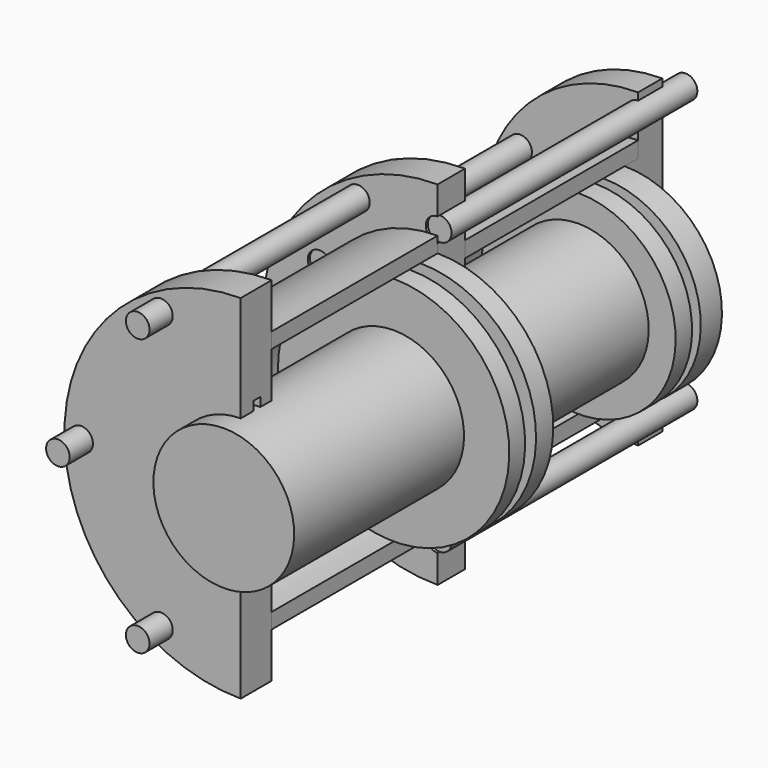
from build123d import *

# Parameters (mm, degrees)
F0_W           = 15.1666663587
F0_H           = 11.4706810564
F8_R           = 3.2667249977
F9_DEPTH       = 77.4214528501
F10_R          = 3.2594816629
F11_DEPTH      = 77.3061978245
F12_DEPTH      = 8
F12_DEPTH_BACK = 83
F13_COUNT      = 6
F14_DEPTH      = 8
F14_DEPTH_BACK = 76.7
F15_COUNT      = 6
F16_W          = 57.5555562973
F16_H          = 106.7500039935
F17_DEPTH      = 100.5891192088
F17_DEPTH_BACK = 60.6954473386


with BuildPart() as f1:
    # F0 (on Right) → F1 (revolve)
    with BuildSketch(Plane.YZ):
        Polygon((-7.1944748051, 11.4706810564), (0, 11.4706810564), (0, 19.4079772794), (-42.000003159, 19.4079772794), (-45.8828173578, 19.4079772794), (-48.3576916158, 19.4079772794), (-52.6944473386, 19.4079772794), (-58.5277788341, 19.4079772794), (-58.5277788341, 0), (-7.1944748051, 0), align=None)
        Polygon((0, 19.4079772794), (0, 11.4706810564), (15.1666663587, 11.4706810564), (15.1666663587, 19.4079772794), (15.1666663587, 31.8888910115), (9.2266909778, 31.8888910115), (9.2266909778, 26.8329977989), (5.4660085589, 26.8329977989), (5.4660085589, 31.8888910115), (0, 31.8888910115), align=None)
    revolve(axis=Axis((0, -29.2638894171, 0), (0, -1, 0)))


with BuildPart() as f2:
    # F0 (on Right) → F2 (revolve)
    with BuildSketch(Plane.YZ):
        Polygon((15.1666663587, 11.4706810564), (15.1666663587, 0), (63.6523626745, 0), (63.6523626745, 19.4079772794), (24.6117504859, 19.4079772794), (21.5158667415, 19.4079772794), (18.2785782963, 19.4079772794), (15.1666663587, 19.4079772794), align=None)
        with Locations((7.5833331794, 5.7353405282)):
            Rectangle(F0_W, F0_H)
        Polygon((63.6523626745, 19.4079772794), (63.6523626745, 0), (79.6123966575, 0), (79.6123966575, 26.8329977989), (72.304725647, 26.8329977989), (72.304725647, 21.5597935021), (69.3202018738, 21.5597935021), (69.3202018738, 26.8329977989), (63.6523626745, 26.8329977989), align=None)
    revolve(axis=Axis((0, 39.4095145166, 0), (0, 1, 0)))


with BuildPart() as f3:
    # F0 (on Right) → F3 (revolve)
    with BuildSketch(Plane.YZ):
        Polygon((-45.8828173578, 19.4079772794), (-42.000003159, 19.4079772794), (-42.000003159, 31.8888910115), (-42.000003159, 36.1666679382), (-42.000003159, 48.611111939), (-52.6944473386, 48.611111939), (-52.6944473386, 19.4079772794), (-48.3576916158, 19.4079772794), (-48.3576916158, 21.8804795295), (-45.8828173578, 21.8804795295), align=None)
    revolve(axis=Axis((0, -29.2638894171, 0), (0, -1, 0)))


with BuildPart() as f4:
    # F0 (on Right) → F4 (revolve)
    with BuildSketch(Plane.YZ):
        Polygon((15.1666663587, 31.8888910115), (15.1666663587, 19.4079772794), (18.2785782963, 19.4079772794), (18.2785782963, 21.8804795295), (21.5158667415, 21.8804795295), (21.5158667415, 19.4079772794), (24.6117504859, 19.4079772794), (24.6117504859, 26.8329977989), (24.6117504859, 31.2296506017), (24.6117504859, 48.611111939), (15.1666663587, 48.611111939), (15.1666663587, 36.1666679382), align=None)
    revolve(axis=Axis((0, 39.4095145166, 0), (0, 1, 0)))


with BuildPart() as f5:
    # F0 (on Right) → F5 (revolve)
    with BuildSketch(Plane.YZ):
        Polygon((79.6123966575, 26.8329977989), (79.6123966575, 0), (82.4770107865, 0), (84.2622816563, 0), (92.5881192088, 0), (92.5881192088, 42.8648870438), (84.2622816563, 42.8648870438), (84.2622816563, 31.2296506017), (84.2622816563, 26.8329977989), align=None)
    revolve(axis=Axis((0, 39.4095145166, 0), (0, 1, 0)))


with BuildPart() as f6:
    # F0 (on Right) → F6 (revolve)
    with BuildSketch(Plane.YZ):
        Polygon((-42.000003159, 31.8888910115), (0, 31.8888910115), (5.4660085589, 31.8888910115), (9.2266909778, 31.8888910115), (15.1666663587, 31.8888910115), (15.1666663587, 36.1666679382), (-42.000003159, 36.1666679382), align=None)
    revolve(axis=Axis((0, -29.2638894171, 0), (0, -1, 0)))


with BuildPart() as f7:
    # F0 (on Right) → F7 (revolve)
    with BuildSketch(Plane.YZ):
        Polygon((72.304725647, 26.8329977989), (79.6123966575, 26.8329977989), (84.2622816563, 26.8329977989), (84.2622816563, 31.2296506017), (24.6117504859, 31.2296506017), (24.6117504859, 26.8329977989), (63.6523626745, 26.8329977989), (69.3202018738, 26.8329977989), align=None)
    revolve(axis=Axis((0, 39.4095145166, 0), (0, 1, 0)))


with BuildPart() as f9_tool:
    # F8 (on face) → F9 (new body, through all)
    with BuildSketch(Plane(origin=(0, 92.5881192088, 0), x_dir=(-1, 0, 0), z_dir=(0, 1, 0))):
        with Locations((-32.5408682228, 18.7874790281)):
            Circle(F8_R)
        with Locations((0, 37.5749580562)):
            Circle(F8_R)
        with Locations((32.5408682228, 18.7874790281)):
            Circle(F8_R)
        with Locations((32.5408682228, -18.7874790281)):
            Circle(F8_R)
        with Locations((0, -37.5749580562)):
            Circle(F8_R)
        with Locations((-32.5408682228, -18.7874790281)):
            Circle(F8_R)
    extrude(amount=-F9_DEPTH)


with BuildPart() as f4_1:
    add(f4.part)

    # F9: cut by f9_tool
    add(f9_tool.part, mode=Mode.SUBTRACT)


with BuildPart() as f5_1:
    add(f5.part)

    # F9: cut by f9_tool
    add(f9_tool.part, mode=Mode.SUBTRACT)


with BuildPart() as f11_tool:
    # F10 (on face) → F11 (new body, through all)
    with BuildSketch(Plane.XZ.offset(52.6944473386)):
        with Locations((-21.9988788281, 38.1031758399)):
            Circle(F10_R)
        with Locations((-43.9977576563, 0)):
            Circle(F10_R)
        with Locations((-21.9988788281, -38.1031758399)):
            Circle(F10_R)
        with Locations((21.9988788281, -38.1031758399)):
            Circle(F10_R)
        with Locations((43.9977576563, 0)):
            Circle(F10_R)
        with BuildLine():
            Line((23.6286196596, 40.9259697631), (20.3691379967, 35.2803819167))
            ThreePointArc((20.3691379967, 35.2803819167), (23.6286196596, 35.2803819167), (25.258360491, 38.1031758399))
            ThreePointArc((25.258360491, 38.1031758399), (24.8216727514, 39.7329166713), (23.6286196596, 40.9259697631))
        make_face()
        with BuildLine():
            ThreePointArc((23.6286196596, 40.9259697631), (19.1760849049, 39.7329166713), (20.3691379967, 35.2803819167))
            Line((20.3691379967, 35.2803819167), (23.6286196596, 40.9259697631))
        make_face()
    extrude(amount=-F11_DEPTH)


with BuildPart() as f3_1:
    add(f3.part)

    # F11: cut by f11_tool
    add(f11_tool.part, mode=Mode.SUBTRACT)


with BuildPart() as f4_2:
    add(f4_1.part)

    # F11: cut by f11_tool
    add(f11_tool.part, mode=Mode.SUBTRACT)


with BuildPart() as f12:
    # F10 (on face) → F12 (new body, two sides)
    with BuildSketch(Plane.XZ.offset(52.6944473386)) as f12_sk:
        with Locations((-21.9988788281, 38.1031758399)):
            Circle(F10_R)
    extrude(amount=F12_DEPTH)
    extrude(f12_sk.sketch, amount=-F12_DEPTH_BACK)


with BuildPart() as f13_1:
    # F13: instance of F12
    add(f12.part.rotate(Axis((0, 39.4095145166, 0), (0, 1, 0)), 1 * 360 / F13_COUNT))


with BuildPart() as f13_2:
    # F13: instance of F12
    add(f12.part.rotate(Axis((0, 39.4095145166, 0), (0, 1, 0)), 2 * 360 / F13_COUNT))


with BuildPart() as f13_3:
    # F13: instance of F12
    add(f12.part.rotate(Axis((0, 39.4095145166, 0), (0, 1, 0)), 3 * 360 / F13_COUNT))


with BuildPart() as f13_4:
    # F13: instance of F12
    add(f12.part.rotate(Axis((0, 39.4095145166, 0), (0, 1, 0)), 4 * 360 / F13_COUNT))


with BuildPart() as f13_5:
    # F13: instance of F12
    add(f12.part.rotate(Axis((0, 39.4095145166, 0), (0, 1, 0)), 5 * 360 / F13_COUNT))


with BuildPart() as f14:
    # F8 (on face) → F14 (new body, two sides)
    with BuildSketch(Plane(origin=(0, 92.5881192088, 0), x_dir=(-1, 0, 0), z_dir=(0, 1, 0))) as f14_sk:
        with Locations((0, 37.5749580562)):
            Circle(F8_R)
    extrude(amount=F14_DEPTH)
    extrude(f14_sk.sketch, amount=-F14_DEPTH_BACK)


with BuildPart() as f15_1:
    # F15: instance of F14
    add(f14.part.rotate(Axis((0, 73.9573221654, 0), (0, 1, 0)), 1 * 360 / F15_COUNT))


with BuildPart() as f15_2:
    # F15: instance of F14
    add(f14.part.rotate(Axis((0, 73.9573221654, 0), (0, 1, 0)), 2 * 360 / F15_COUNT))


with BuildPart() as f15_3:
    # F15: instance of F14
    add(f14.part.rotate(Axis((0, 73.9573221654, 0), (0, 1, 0)), 3 * 360 / F15_COUNT))


with BuildPart() as f15_4:
    # F15: instance of F14
    add(f14.part.rotate(Axis((0, 73.9573221654, 0), (0, 1, 0)), 4 * 360 / F15_COUNT))


with BuildPart() as f15_5:
    # F15: instance of F14
    add(f14.part.rotate(Axis((0, 73.9573221654, 0), (0, 1, 0)), 5 * 360 / F15_COUNT))


with BuildPart() as f17_tool:
    # F16 (on Front) → F17 (new body, two sides)
    with BuildSketch(Plane.XZ) as f17_sk:
        with Locations((28.7777781487, 0.6805546582)):
            Rectangle(F16_W, F16_H)
    extrude(amount=-F17_DEPTH)
    extrude(f17_sk.sketch, amount=F17_DEPTH_BACK)


with BuildPart() as f3_2:
    add(f3_1.part)

    # F17: cut by f17_tool
    add(f17_tool.part, mode=Mode.SUBTRACT)


with BuildPart() as f4_3:
    add(f4_2.part)

    # F17: cut by f17_tool
    add(f17_tool.part, mode=Mode.SUBTRACT)


with BuildPart() as f5_2:
    add(f5_1.part)

    # F17: cut by f17_tool
    add(f17_tool.part, mode=Mode.SUBTRACT)


with BuildPart() as f6_1:
    add(f6.part)

    # F17: cut by f17_tool
    add(f17_tool.part, mode=Mode.SUBTRACT)


with BuildPart() as f7_1:
    add(f7.part)

    # F17: cut by f17_tool
    add(f17_tool.part, mode=Mode.SUBTRACT)


with BuildPart() as f13_1_1:
    add(f13_1.part)

    # F17: cut by f17_tool
    add(f17_tool.part, mode=Mode.SUBTRACT)


with BuildPart() as f13_2_1:
    add(f13_2.part)

    # F17: cut by f17_tool
    add(f17_tool.part, mode=Mode.SUBTRACT)


with BuildPart() as f13_3_1:
    add(f13_3.part)

    # F17: cut by f17_tool
    add(f17_tool.part, mode=Mode.SUBTRACT)


with BuildPart() as f15_1_1:
    add(f15_1.part)

    # F17: cut by f17_tool
    add(f17_tool.part, mode=Mode.SUBTRACT)


with BuildPart() as f15_2_1:
    add(f15_2.part)

    # F17: cut by f17_tool
    add(f17_tool.part, mode=Mode.SUBTRACT)


solid = Compound([f1.part, f2.part, f12.part, f13_4.part, f13_5.part, f14.part, f15_3.part, f15_4.part, f15_5.part, f3_2.part, f4_3.part, f5_2.part, f6_1.part, f7_1.part])
